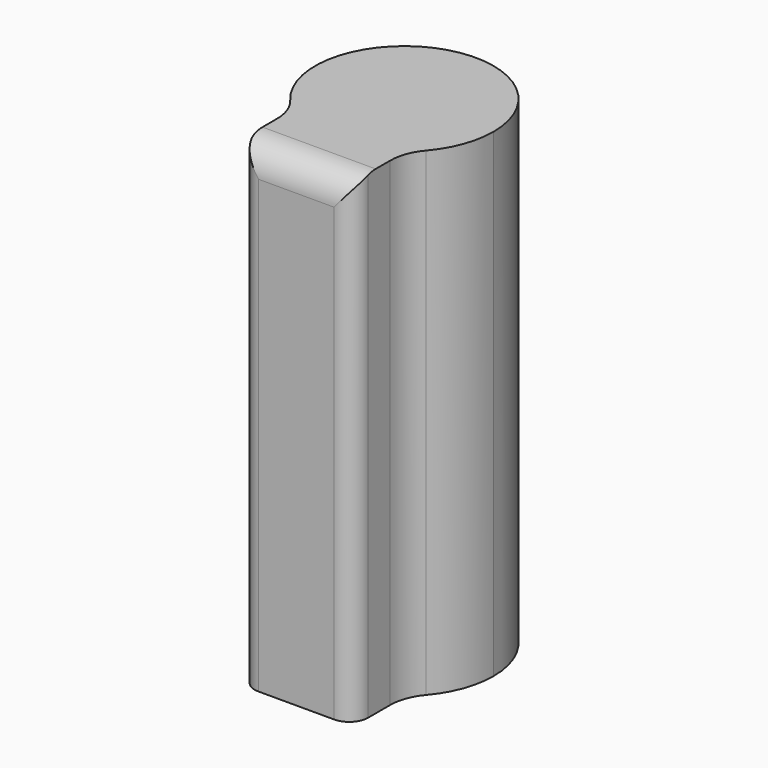
from build123d import *

# Parameters (mm, degrees)
F1_DEPTH    = 50.8
F2_R        = 2
F3_R        = 5
F4_T1_DEPTH = 23


# Not quite as in the source:
# - a fillet or chamfer that OpenCascade refuses, or shapes differently, is made with other operations: its cross-section is extruded or revolved along the edge and cut away or added


with BuildPart() as f1:
    # F0 (on Top) → F1 (new body)
    with BuildSketch(Plane.XY):
        with BuildLine():
            ThreePointArc((6, -7.3008561142), (8.5440768957, -4.0374806501), (9.45, 0))
            ThreePointArc((9.45, 0), (-4.0374806501, 8.5440768957), (-6, -7.3008561142))
            ThreePointArc((-6, -7.3008561142), (0, -9.45), (6, -7.3008561142))
        make_face()
        with BuildLine():
            ThreePointArc((6, -7.3008561142), (0, -9.45), (-6, -7.3008561142))
            Line((-6, -7.3008561142), (-6, -14.3008561142))
            Line((-6, -14.3008561142), (0, -14.3008561142))
            Line((0, -14.3008561142), (6, -14.3008561142))
            Line((6, -14.3008561142), (6, -7.3008561142))
        make_face()
    extrude(amount=F1_DEPTH)

    # F2
    f2_edges = [f1.edges().sort_by_distance(p)[0] for p in [
        (6, -14.300856, 25.4),
        (-6, -14.300856, 25.4),
    ]]
    fillet(f2_edges, radius=F2_R)

    # F3
    f3_edges = [f1.edges().sort_by_distance(p)[0] for p in [
        (-6, -7.300856, 25.4),
        (6, -7.300856, 25.4),
    ]]
    fillet(f3_edges, radius=F3_R)

    # F4: fillet of radius 3 on 1 edges, made by hand

    # F4_s2 → F4_t1 (cut)
    with BuildSketch(Plane.YZ.offset(-11.5)):
        with BuildLine():
            ThreePointArc((-11.3008561142, 50.8), (-13.4221764577, 49.9213203436), (-14.3008561142, 47.8))
            Line((-14.3008561142, 47.8), (-14.3008561142, 50.8))
            Line((-14.3008561142, 50.8), (-11.3008561142, 50.8))
        make_face()
    extrude(amount=F4_T1_DEPTH, mode=Mode.SUBTRACT)


solid = f1.part
